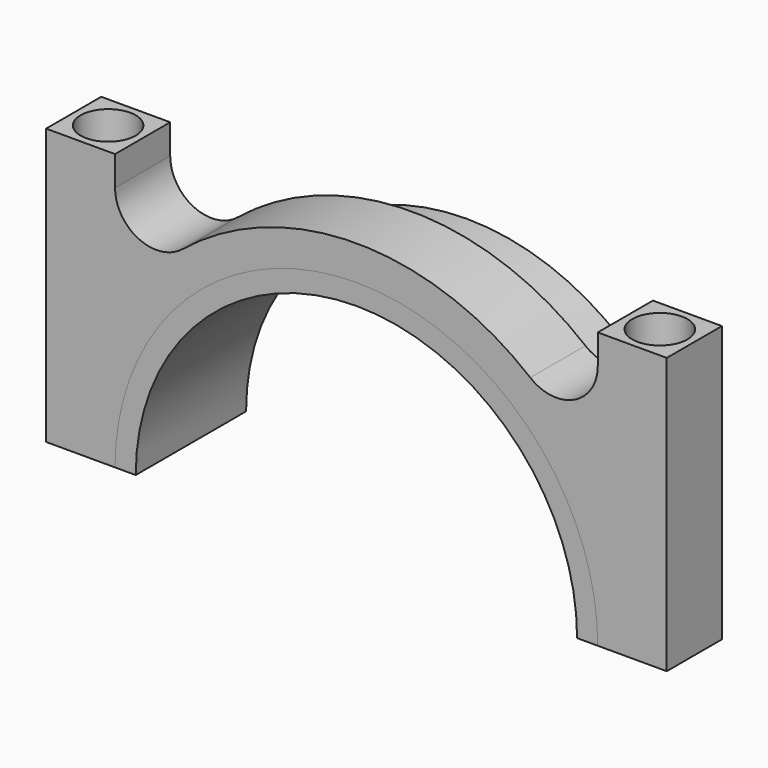
from build123d import *

# Parameters (mm, degrees)
F1_DEPTH = 5
F2_R     = 2
F3_DEPTH = 20.001
F5_DEPTH = 5


# Not quite as in the source:
# - a pattern or mirror of a feature is missing from the dataset's text; its kind, count and spacing are read off the source's solid


with BuildPart() as f1:
    # F0 (on Front) → F1 (new body)
    with BuildSketch(Plane.XZ):
        with BuildLine():
            ThreePointArc((-17.5, 0), (0, 17.5), (17.5, 0))
            Line((17.5, 0), (22.5, 0))
            Line((22.5, 0), (22.5, 20))
            Line((22.5, 20), (17.5, 20))
            Line((17.5, 20), (17.5, 17.8535710714))
            ThreePointArc((17.5, 17.8535710714), (15.7895904304, 15.1448893769), (12.6086956522, 15.5248444099))
            ThreePointArc((12.6086956522, 15.5248444099), (0, 20), (-12.6086956522, 15.5248444099))
            ThreePointArc((-12.6086956522, 15.5248444099), (-15.7895904304, 15.1448893769), (-17.5, 17.8535710714))
            Line((-17.5, 17.8535710714), (-17.5, 20))
            Line((-17.5, 20), (-22.5, 20))
            Line((-22.5, 20), (-22.5, 0))
            Line((-22.5, 0), (-17.5, 0))
        make_face()
    extrude(amount=F1_DEPTH)

    # F2 (on face) → F3 (cut, through all)
    with BuildSketch(Plane.XY.offset(20)):
        with Locations((-20, -2.5)):
            Circle(F2_R)
    f3 = extrude(amount=-F3_DEPTH, mode=Mode.SUBTRACT)

    # F3_copies: F3 across plane
    add(f3.mirror(Plane(origin=(0, 0, 0), x_dir=(0, 0, 1), z_dir=(1, 0, 0))), mode=Mode.SUBTRACT)


with BuildPart() as f5:
    # F4 (on Front) → F5 (new body, symmetric)
    with BuildSketch(Plane.XZ):
        with BuildLine():
            ThreePointArc((-16, 0), (0, 16), (16, 0))
            Line((16, 0), (17.5, 0))
            ThreePointArc((17.5, 0), (0, 17.5), (-17.5, 0))
            Line((-17.5, 0), (-16, 0))
        make_face()
    extrude(amount=F5_DEPTH, both=True)


solid = Compound([f1.part, f5.part])
